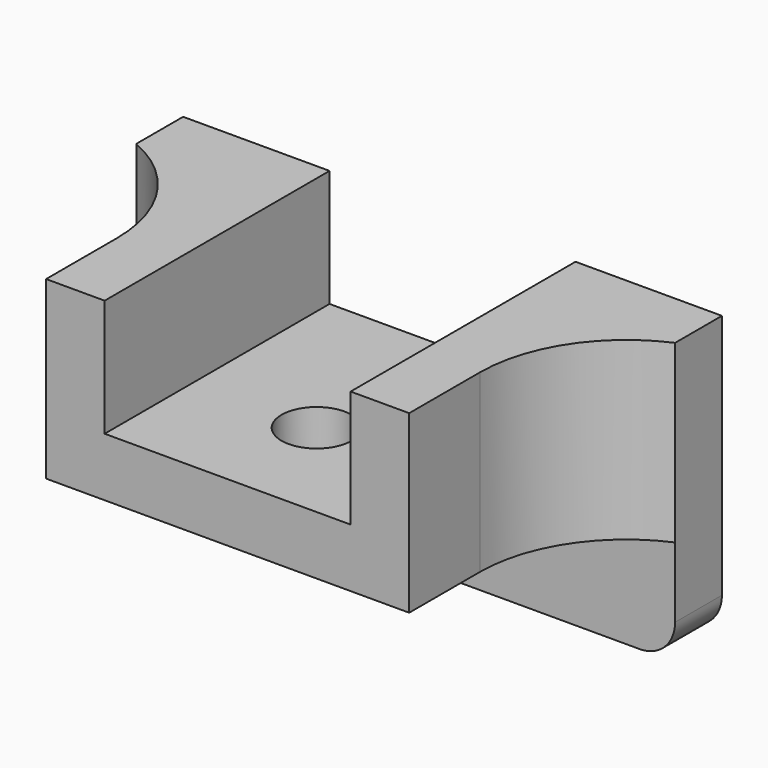
from build123d import *

# Parameters (mm, degrees)
F1_DEPTH    = 48
F2_DEPTH    = 10
F3_R        = 6
F4_DEPTH    = 3
F5_DEPTH    = 5
F6_T1_DEPTH = 30
F7_D        = 12


# Not quite as in the source:
# - a fillet or chamfer that OpenCascade refuses, or shapes differently, is made with other operations: its cross-section is extruded or revolved along the edge and cut away or added


with BuildPart() as f1:
    # F0 (on Front) → F1 (new body)
    with BuildSketch(Plane.XZ):
        Polygon((-21, 0), (-31, 0), (-31, -30), (31, -30), (31, 0), (21, 0), (21, -20), (-21, -20), align=None)
    extrude(amount=F1_DEPTH)

    # F0 (on Front) → F2 (join)
    with BuildSketch(Plane.XZ):
        with BuildLine():
            Line((-31, 0), (-46, 0))
            Line((-46, 0), (-46, -42))
            ThreePointArc((-46, -42), (-44.2426406871, -46.2426406871), (-40, -48))
            Line((-40, -48), (40, -48))
            ThreePointArc((40, -48), (44.2426406871, -46.2426406871), (46, -42))
            Line((46, -42), (46, 0))
            Line((46, 0), (31, 0))
            Line((31, 0), (31, -30))
            Line((31, -30), (-31, -30))
            Line((-31, -30), (-31, 0))
        make_face()
        Polygon((-21, 0), (-31, 0), (-31, -30), (31, -30), (31, 0), (21, 0), (21, -20), (-21, -20), align=None)
    extrude(amount=F2_DEPTH)

    # F3 (on face) → F4 (join)
    with BuildSketch(Plane(origin=(0, 0, -30), x_dir=(1, 0, 0), z_dir=(0, 0, -1))):
        with BuildLine():
            Line((13.9955899146, 15), (13.9955899146, 28.6486270591))
            ThreePointArc((13.9955899146, 28.6486270591), (0.0417417441, 42.9999377722), (-13.9974363474, 28.7320901258))
            Line((-13.9974363474, 28.7320901258), (-13.7346051799, 15))
            Line((-13.7346051799, 15), (13.9955899146, 15))
        make_face()
        with Locations((0, 29)):
            Circle(F3_R, mode=Mode.SUBTRACT)
    extrude(amount=F4_DEPTH)

    # F3 (on face) → F5 (join)
    with BuildSketch(Plane(origin=(0, 0, -30), x_dir=(1, 0, 0), z_dir=(0, 0, -1))):
        Polygon((13.9955899146, 10), (13.9955899146, 15), (-13.7346051799, 15), (-13.6389055576, 10), align=None)
    extrude(amount=F5_DEPTH)

    # F6: fillet of radius 25 on 2 edges, made by hand

    # F6_s2 → F6_t1 (join)
    with BuildSketch(Plane.XY.offset(-30)):
        with BuildLine():
            ThreePointArc((31, -32.9128784748), (35.0834993366, -19.2198145372), (46, -10))
            Line((46, -10), (31, -10))
            Line((31, -10), (31, -32.9128784748))
        make_face()
        with BuildLine():
            ThreePointArc((-46, -10), (-35.0834993366, -19.2198145372), (-31, -32.9128784748))
            Line((-31, -32.9128784748), (-31, -10))
            Line((-31, -10), (-46, -10))
        make_face()
    extrude(amount=F6_T1_DEPTH)

    # F7 (through all)
    with Locations(Plane(origin=(0, 0, -30), x_dir=(1, 0, 0), z_dir=(0, 0, -1))):
        with Locations((0, 29)):
            Hole(F7_D / 2)


solid = f1.part
